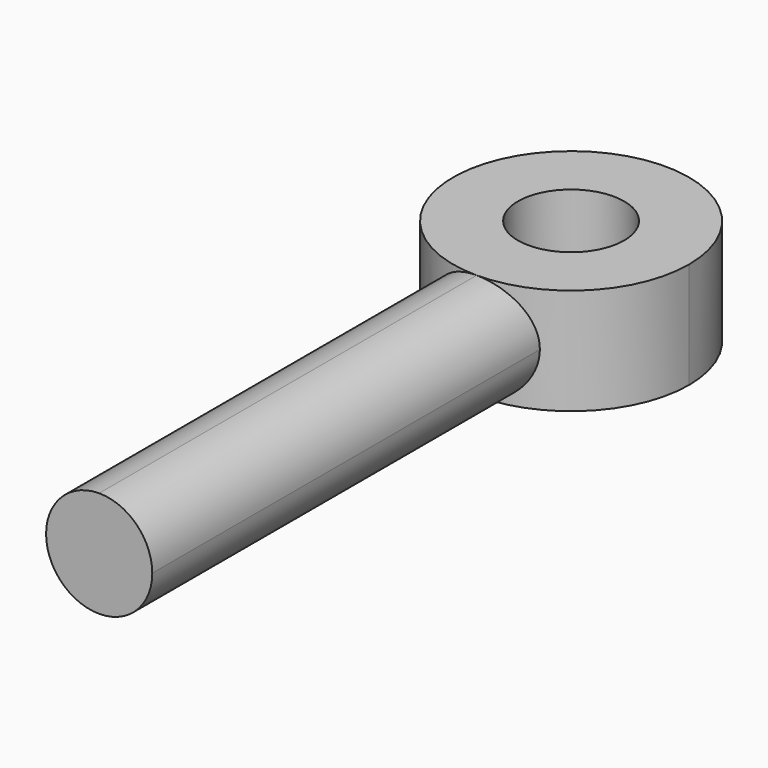
from build123d import *

# Parameters (mm, degrees)
F1_DEPTH = 9
F2_R     = 4.49999


# Not quite as in the source:
# - a fillet or chamfer is up to 0.001 mm smaller than in the source, because OpenCascade refuses the exact size


with BuildPart() as f1:
    # F0 (on Top) → F1 (new body)
    with BuildSketch(Plane.XY):
        with BuildLine():
            ThreePointArc((4.5, -8.9302855497), (8.514693183, -5.2440442409), (10, 0))
            ThreePointArc((10, 0), (-5.2440442409, 8.514693183), (-4.5, -8.9302855497))
            Line((-4.5, -8.9302855497), (-4.5, 0))
            ThreePointArc((-4.5, 0), (0, 4.5), (4.5, 0))
            Line((4.5, 0), (4.5, -8.9302855497))
        make_face()
        with BuildLine():
            Line((-4.5, 0), (-4.5, -8.9302855497))
            ThreePointArc((-4.5, -8.9302855497), (0, -10), (4.5, -8.9302855497))
            Line((4.5, -8.9302855497), (4.5, 0))
            ThreePointArc((4.5, 0), (0, -4.5), (-4.5, 0))
        make_face()
        with BuildLine():
            ThreePointArc((4.5, -8.9302855497), (0, -10), (-4.5, -8.9302855497))
            Line((-4.5, -8.9302855497), (-4.5, -50))
            Line((-4.5, -50), (4.5, -50))
            Line((4.5, -50), (4.5, -8.9302855497))
        make_face()
    extrude(amount=F1_DEPTH)

    # F2 (radius 4.5 in the source; OpenCascade refuses exactly that, so slightly less here)
    f2_edges = [f1.edges().sort_by_distance(p)[0] for p in [
        (-4.5, -29.465143, 9),
        (4.5, -29.465143, 9),
        (4.5, -29.465143, 0),
        (-4.5, -29.465143, 0),
    ]]
    fillet(f2_edges, radius=F2_R)


solid = f1.part
